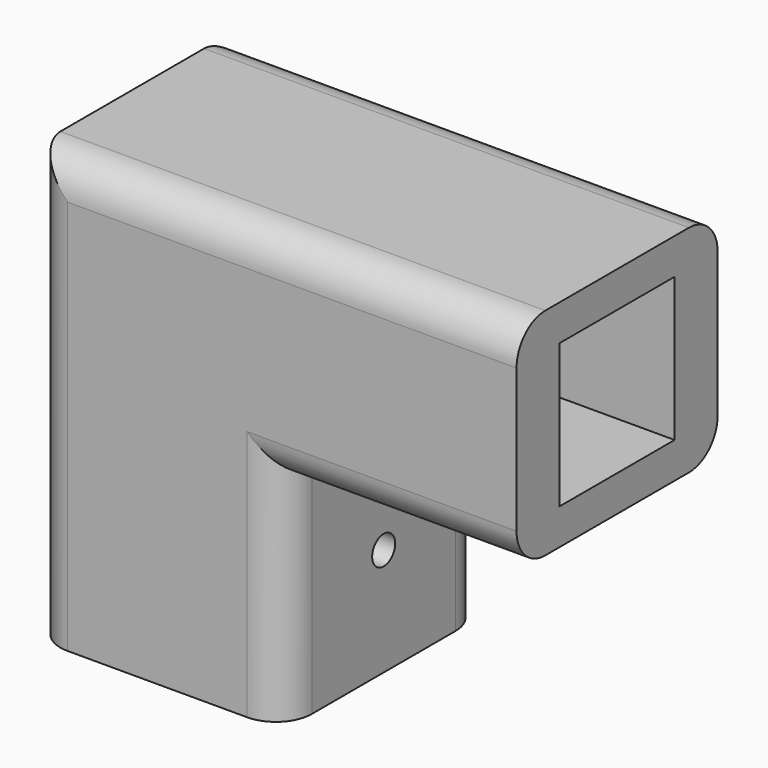
from build123d import *

# Parameters (mm, degrees)
F0_W      = 35
F0_H      = 35
F0_W_2    = 20
F0_H_2    = 20
F1_DEPTH  = 60
F3_R      = 2
F4_DEPTH  = 10
F6_W      = 35
F6_H      = 30
F6_W_2    = 20
F6_H_2    = 20
F7_DEPTH  = 50
F8_DEPTH  = 17.5
F9_DEPTH  = 60
F10_DEPTH = 10.25
F11_DEPTH = 55
F12_R     = 5
F13_R     = 2
F14_DEPTH = 20


# Not quite as in the source:
# - a feature of the source that left no trace in its solid (it failed there, or was rolled back) is left out


with BuildPart() as f1:
    # F0 (on Top) → F1 (new body)
    with BuildSketch(Plane.XY):
        Rectangle(F0_W, F0_H)
        Rectangle(F0_W_2, F0_H_2, mode=Mode.SUBTRACT)
    extrude(amount=F1_DEPTH)

    # F3 (on face) → F4 (cut)
    with BuildSketch(Plane.YZ.offset(17.5)):
        with Locations((0, 40)):
            Circle(F3_R)
        with Locations((0, 15)):
            Circle(F3_R)
    extrude(amount=-F4_DEPTH, mode=Mode.SUBTRACT)

    # F6 (on Right) → F7 (join)
    with BuildSketch(Plane.YZ):
        with Locations((0, 45)):
            Rectangle(F6_W, F6_H)
        with Locations((0, 45)):
            Rectangle(F6_W_2, F6_H_2, mode=Mode.SUBTRACT)
        with Locations((0, 45)):
            Rectangle(F6_W_2, F6_H_2)
    extrude(amount=F7_DEPTH)

    # F6 (on Right) → F8 (join, through all)
    with BuildSketch(Plane.YZ):
        with Locations((0, 45)):
            Rectangle(F6_W, F6_H)
        with Locations((0, 45)):
            Rectangle(F6_W_2, F6_H_2, mode=Mode.SUBTRACT)
        with Locations((0, 45)):
            Rectangle(F6_W_2, F6_H_2)
    extrude(amount=-F8_DEPTH)

    # F6 (on Right) → F9 (cut)
    with BuildSketch(Plane.YZ):
        with Locations((0, 45)):
            Rectangle(F6_W_2, F6_H_2)
    extrude(amount=F9_DEPTH, mode=Mode.SUBTRACT)

    # F6 (on Right) → F10 (cut)
    with BuildSketch(Plane.YZ):
        with Locations((0, 45)):
            Rectangle(F6_W_2, F6_H_2)
    extrude(amount=-F10_DEPTH, mode=Mode.SUBTRACT)

    # F0 (on Top) → F11 (cut, through all)
    with BuildSketch(Plane.XY):
        Rectangle(F0_W_2, F0_H_2)
    extrude(amount=F11_DEPTH, mode=Mode.SUBTRACT)

    # F12
    f12_edges = [f1.edges().sort_by_distance(p)[0] for p in [
        (-17.5, -17.5, 30),
        (-17.5, 17.5, 30),
        (33.75, -17.5, 30),
        (33.75, 17.5, 30),
        (16.25, 17.5, 60),
        (16.25, -17.5, 60),
        (17.5, -17.5, 15),
        (17.5, 17.5, 15),
    ]]
    fillet(f12_edges, radius=F12_R)

    # F13 (on face) → F14 (cut)
    with BuildSketch(Plane(origin=(0, 0, 30), x_dir=(1, 0, 0), z_dir=(0, 0, -1))):
        with Locations((35, 0)):
            Circle(F13_R)
    extrude(amount=-F14_DEPTH, mode=Mode.SUBTRACT)


solid = f1.part
